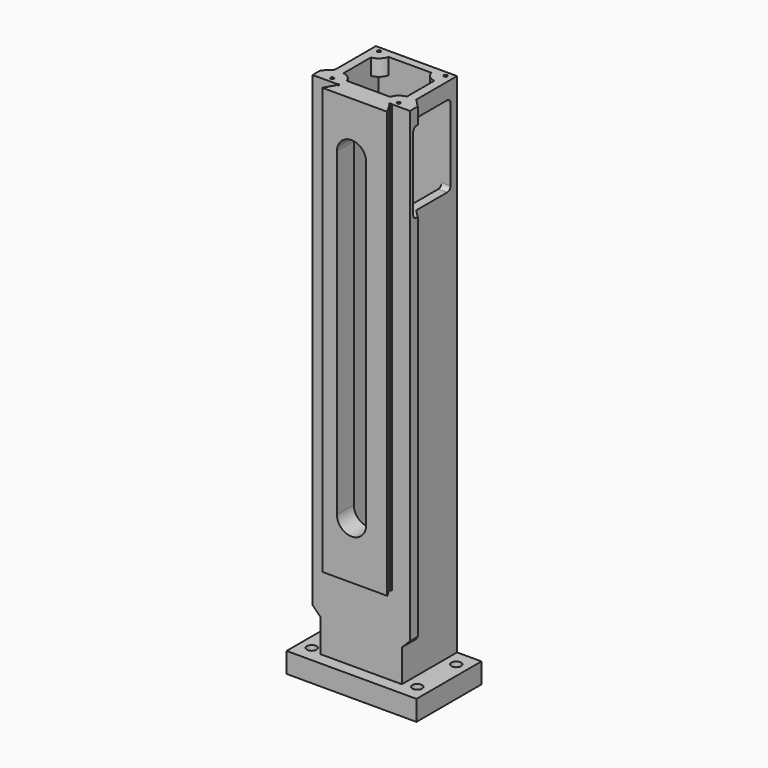
from build123d import *

# Parameters (mm, degrees)
F0_W           = 160
F0_H           = 100
F0_R           = 6
F0_W_2         = 78
F0_H_2         = 64
F1_DEPTH       = 25
F2_W           = 78
F2_H           = 64
F3_DEPTH       = 625
F5_DEPTH       = 26
F6_W           = 80
F6_H           = 100
F7_DEPTH       = 15
F9_DEPTH       = 22
F11_D          = 4.2
F11_DEPTH      = 10.4
F11_TIP        = 1.2618073
F13_DEPTH      = 20
F15_DEPTH      = 21
F17_DEPTH      = 525
F17_DEPTH_BACK = 3
F18_R          = 1.24999


# Not quite as in the source:
# - a fillet or chamfer is up to 0.001 mm smaller than in the source, because OpenCascade refuses the exact size


with BuildPart() as f1:
    # F0 (on Top) → F1 (new body)
    with BuildSketch(Plane.XY):
        Rectangle(F0_W, F0_H)
        with Locations((-65, -30)):
            Circle(F0_R, mode=Mode.SUBTRACT)
        with Locations((65, -30)):
            Circle(F0_R, mode=Mode.SUBTRACT)
        with Locations((-65, 30)):
            Circle(F0_R, mode=Mode.SUBTRACT)
        with Locations((0, 8)):
            Rectangle(F0_W_2, F0_H_2, mode=Mode.SUBTRACT)
        with Locations((65, 30)):
            Circle(F0_R, mode=Mode.SUBTRACT)
    extrude(amount=F1_DEPTH)

    # F2 (on face) → F3 (join)
    with BuildSketch(Plane.XY.offset(25)):
        Polygon((50, 50), (-50, 50), (-50, -13), (-60, -23), (-60, -35), (-27.3397459622, -35), (-36, -50), (44, -50), (35.3397459622, -35), (60, -35), (60, -23), (50, -13), align=None)
        with Locations((0, 8)):
            Rectangle(F2_W, F2_H, mode=Mode.SUBTRACT)
    extrude(amount=F3_DEPTH)

    # F4 (on face) → F5 (cut, through all)
    with BuildSketch(Plane.XZ.offset(50)):
        with BuildLine():
            ThreePointArc((-18, 193), (0, 175), (18, 193))
            Line((18, 193), (18, 587))
            ThreePointArc((18, 587), (0, 605), (-18, 587))
            Line((-18, 587), (-18, 193))
        make_face()
    extrude(amount=-F5_DEPTH, mode=Mode.SUBTRACT)

    # F6 (on face) → F7 (cut, through all)
    with BuildSketch(Plane.XZ.offset(50)):
        with Locations((4, 75)):
            Rectangle(F6_W, F6_H)
    extrude(amount=-F7_DEPTH, mode=Mode.SUBTRACT)

    # F8 (on face) → F9 (cut, through all)
    with BuildSketch(Plane.XZ.offset(35)):
        Polygon((-60, 75), (-60, 25), (-50, 25), (-50, 65), align=None)
        Polygon((50, 65), (50, 25), (60, 25), (60, 75), align=None)
    extrude(amount=-F9_DEPTH, mode=Mode.SUBTRACT)

    # F11
    with Locations(Plane.XY.offset(650)):
        with Locations((-41, 43.5), (41, 43.5), (41, -28.5), (-41, -28.5)):
            Hole(F11_D / 2, depth=F11_DEPTH)
            with Locations((0, 0, -(F11_DEPTH + F11_TIP / 2))):  # 118° drill point
                Cone(0, F11_D / 2, F11_TIP, mode=Mode.SUBTRACT)

    # F12 (on face) → F13 (join)
    with BuildSketch(Plane.XY.offset(650)):
        with BuildLine():
            Line((-39, 40), (-39, 28.6339312527))
            ThreePointArc((-39, 28.6339312527), (-30.9466258481, 32.367629715), (-26.4140478542, 40))
            Line((-26.4140478542, 40), (-39, 40))
        make_face()
        with BuildLine():
            Line((39, 40), (26.4140478542, 40))
            ThreePointArc((26.4140478542, 40), (30.9466258481, 32.367629715), (39, 28.6339312527))
            Line((39, 28.6339312527), (39, 40))
        make_face()
        with BuildLine():
            ThreePointArc((-26.6909119787, -24), (-31.3376797124, -17.0265712771), (-39, -13.6339312527))
            Line((-39, -13.6339312527), (-39, -24))
            Line((-39, -24), (-26.6909119787, -24))
        make_face()
        with BuildLine():
            ThreePointArc((39, -13.6339312527), (31.3376797124, -17.0265712771), (26.6909119787, -24))
            Line((26.6909119787, -24), (39, -24))
            Line((39, -24), (39, -13.6339312527))
        make_face()
    extrude(amount=-F13_DEPTH)

    # F14 (on face) → F15 (cut, through all)
    with BuildSketch(Plane.YZ.offset(60)):
        with BuildLine():
            Line((35, 630), (-23, 630))
            Line((-23, 630), (-23, 530))
            Line((-23, 530), (35, 530))
            ThreePointArc((35, 530), (38.5355339059, 531.4644660941), (40, 535))
            Line((40, 535), (40, 625))
            ThreePointArc((40, 625), (38.5355339059, 628.5355339059), (35, 630))
        make_face()
        with BuildLine():
            Line((-23, 630), (-25, 630))
            ThreePointArc((-25, 630), (-28.5355339059, 628.5355339059), (-30, 625))
            Line((-30, 625), (-30, 535))
            ThreePointArc((-30, 535), (-28.5355339059, 531.4644660941), (-25, 530))
            Line((-25, 530), (-23, 530))
            Line((-23, 530), (-23, 630))
        make_face()
    extrude(amount=-F15_DEPTH, mode=Mode.SUBTRACT)

    # F16 (on face) → F17 (cut, two sides)
    with BuildSketch(Plane(origin=(0, 0, 125), x_dir=(1, 0, 0), z_dir=(0, 0, -1))) as f17_sk:
        Polygon((36.5897459622, 37.1650635095), (34.7147459622, 36.0825317547), (35.9647459622, 33.9174682453), (37.8397459622, 35), align=None)
        Polygon((-27.9647459622, 33.9174682453), (-26.7147459622, 36.0825317547), (-28.5897459622, 37.1650635095), (-29.8397459622, 35), align=None)
    extrude(amount=-F17_DEPTH, mode=Mode.SUBTRACT)
    extrude(f17_sk.sketch, amount=F17_DEPTH_BACK, mode=Mode.SUBTRACT)

    # F18 (radius 1.25 in the source; OpenCascade refuses exactly that, so slightly less here)
    f18_edges = [f1.edges().sort_by_distance(p)[0] for p in [
        (36.902246, -34.458734, 122),
        (-28.902246, -34.458734, 122),
    ]]
    fillet(f18_edges, radius=F18_R)


solid = f1.part
